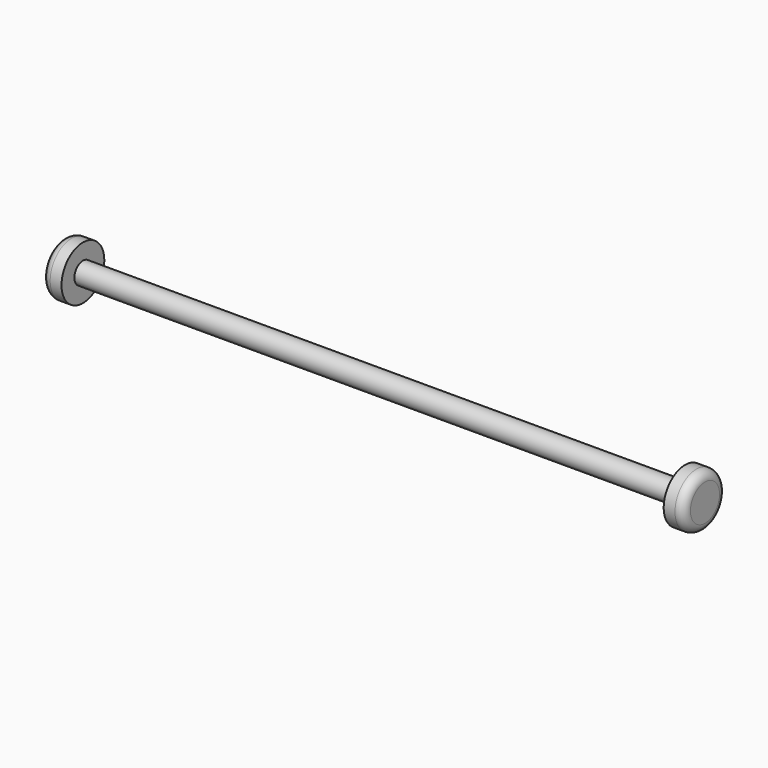
from build123d import *

# Parameters (mm, degrees)
F0_W   = 1.85994
F0_H   = 1
F0_H_2 = 1.5
F2_R   = 0.8


with BuildPart() as f1:
    # F0 (on Front) → F1 (revolve)
    with BuildSketch(Plane.XZ):
        Polygon((-28.14006, 0), (0, 0), (28.14006, 0), (28.14006, 1), (-28.14006, 1), align=None)
        with Locations((29.07003, -0.5)):
            Rectangle(F0_W, F0_H)
        with Locations((-29.07003, 0.5)):
            Rectangle(F0_W, F0_H)
        with Locations((29.07003, 1.75)):
            Rectangle(F0_W, F0_H_2)
        with Locations((-29.07003, 1.75)):
            Rectangle(F0_W, F0_H_2)
    revolve(axis=Axis((0, 0, 0), (-1, 0, 0)))

    # F2
    f2_edges = [f1.edges().sort_by_distance(p)[0] for p in [
        (-30, 0, -2.5),
        (30, 0, -2.5),
    ]]
    fillet(f2_edges, radius=F2_R)


solid = f1.part
